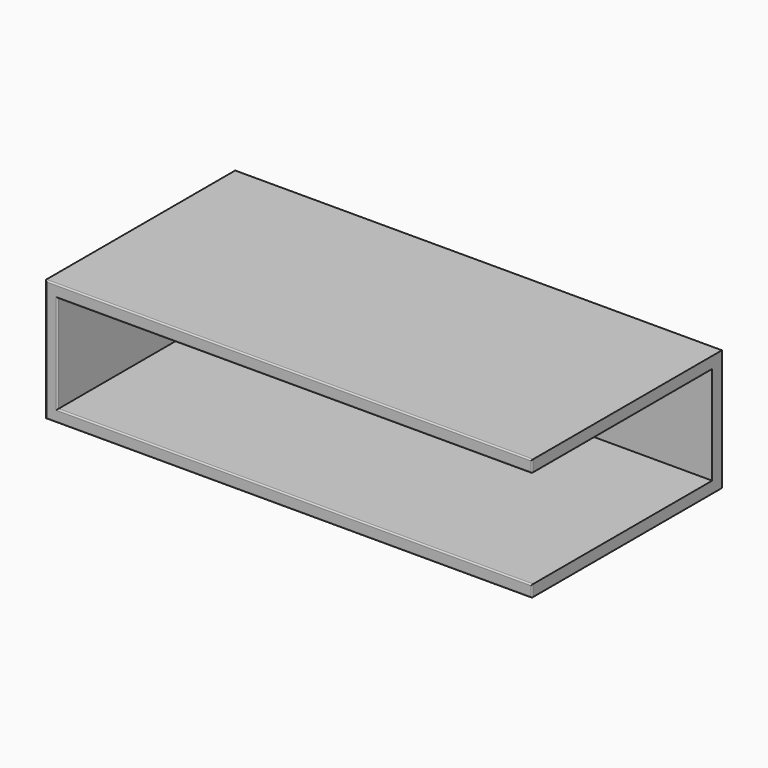
from build123d import *

# Parameters (mm, degrees)
F0_W     = 51.6054928303
F0_H     = 42.5849854946
F1_DEPTH = 350
F2_DEPTH = 718
F3_DEPTH = 180
F4_T     = -18
F5_R     = 2


# Not quite as in the source:
# - two fillets or chamfers of one size are made in one step


with BuildPart() as f1:
    # F0 (on Front) → F1 (new body)
    with BuildSketch(Plane.XZ):
        with Locations((25.8027464151, 21.2924927473)):
            Rectangle(F0_W, F0_H)
    extrude(amount=F1_DEPTH)

    # F2 (add): a face of the model
    f2_faces = [f1.faces().sort_by_distance(p)[0] for p in [
        (0, -175, 21.2924927473),
    ]]
    extrude(f2_faces, amount=-F2_DEPTH)

    # F3 (add): a face of the model
    f3_faces = [f1.faces().sort_by_distance(p)[0] for p in [
        (359, -175, 0),
    ]]
    extrude(f3_faces, amount=-F3_DEPTH)

    # F4
    f4_openings = [f1.faces().sort_by_distance(p)[0] for p in [
        (359, -350, 90),
        (718, -175, 90),
    ]]
    offset(amount=F4_T, openings=f4_openings)

    # F5
    f5_edges = [f1.edges().sort_by_distance(p)[0] for p in [
        (359, -350, 180),
        (0, -350, 90),
        (359, -350, 0),
        (718, -175, 0),
        (718, -350, 9),
        (368, -350, 18),
        (18, -350, 90),
        (368, -350, 162),
        (718, -350, 171),
        (718, -184, 162),
    ]]
    fillet(f5_edges, radius=F5_R)


solid = f1.part
